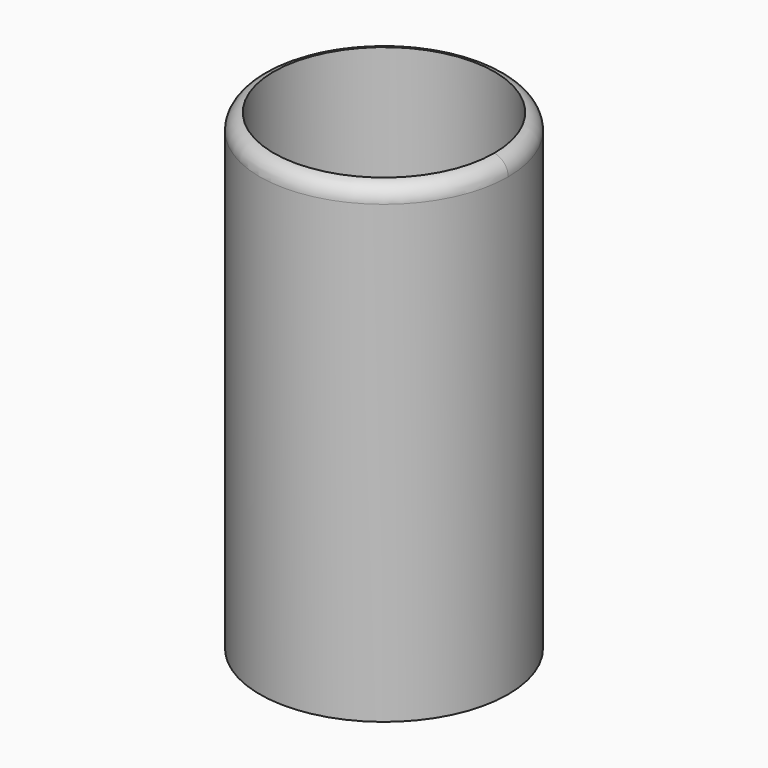
from build123d import *

# Parameters (mm, degrees)
F0_R        = 38.1
F1_DEPTH    = 20.32
F2_R        = 38.1
F3_DEPTH    = 124.46
F5_DEPTH    = 122.682
F6_T2_ANGLE = 179.9999997765
F6_T4_ANGLE = 180.0000002235


# Not quite as in the source:
# - a fillet or chamfer that OpenCascade refuses, or shapes differently, is made with other operations: its cross-section is extruded or revolved along the edge and cut away or added
# - a feature names something its author has since deleted; it is built from what else it names


with BuildPart() as f1:
    # F0 (on Top) → F1 (new body)
    with BuildSketch(Plane.XY):
        Circle(F0_R)
    extrude(amount=F1_DEPTH)

    # F2 (on face) → F3 (join)
    with BuildSketch(Plane.XY.offset(20.32)):
        Circle(F2_R)
    extrude(amount=F3_DEPTH)

    # F4 (on face) → F5 (cut, symmetric)
    with BuildSketch(Plane.XY.offset(144.78)):
        with BuildLine():
            ThreePointArc((-33.8414182484, 0), (0, -33.8414182484), (33.8414182484, 0))
            ThreePointArc((33.8414182484, 0), (0, 33.8414182484), (-33.8414182484, 0))
        make_face()
    extrude(amount=F5_DEPTH, both=True, mode=Mode.SUBTRACT)

    # F6: fillet of radius 5.08 on 1 edges, made by hand

    # F6_s1 → F6_t2 (revolve, cut)
    with BuildSketch(Plane.XZ):
        with BuildLine():
            ThreePointArc((38.1, 139.7668500859), (36.8916407828, 143.0557401189), (33.8414182484, 144.78))
            Line((33.8414182484, 144.78), (38.1, 144.78))
            Line((38.1, 144.78), (38.1, 139.7668500859))
        make_face()
    revolve(axis=Axis((0, 0, 144.78), (0, 0, 1)), revolution_arc=F6_T2_ANGLE, mode=Mode.SUBTRACT)

    # F6_s3 → F6_t4 (revolve, cut)
    with BuildSketch(Plane.XZ):
        with BuildLine():
            ThreePointArc((-38.1, 139.7668500859), (-36.8916407828, 143.0557401189), (-33.8414182484, 144.78))
            Line((-33.8414182484, 144.78), (-38.1, 144.78))
            Line((-38.1, 144.78), (-38.1, 139.7668500859))
        make_face()
    revolve(axis=Axis((0, 0, 144.78), (0, 0, 1)), revolution_arc=F6_T4_ANGLE, mode=Mode.SUBTRACT)


solid = f1.part
